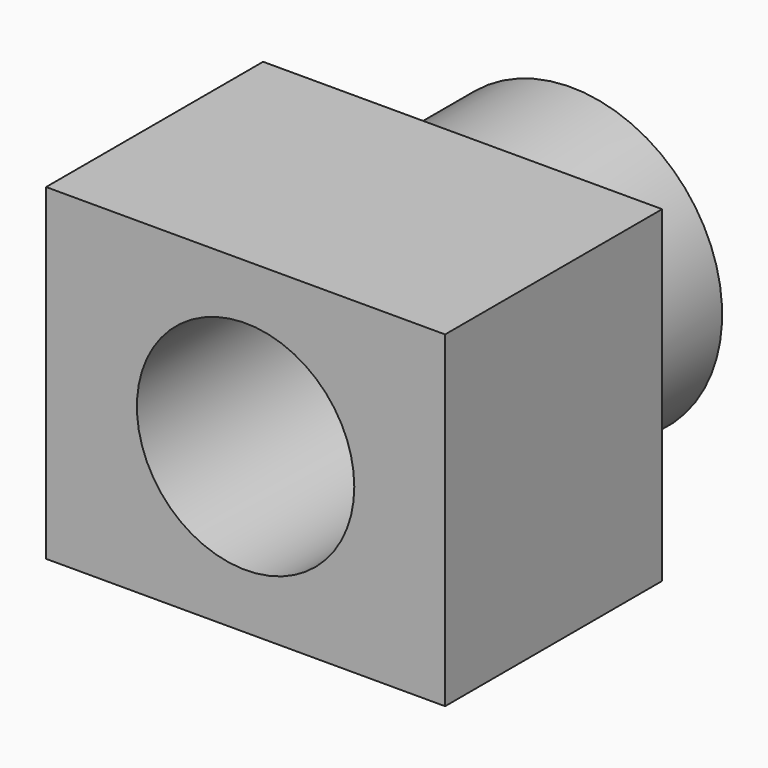
from build123d import *
from build123d import SkipClean  # not in build123d's __all__

# Parameters (mm, degrees)
F0_W     = 74.7220367193
F0_H     = 61.2964034081
F1_DEPTH = 25.4
F2_R     = 20.3537507695
F3_DEPTH = 50.801
F4_R     = 28.2811450825
F4_R_2   = 20.3537507695
F5_DEPTH = 25.4


with BuildPart() as f1:
    # F0 (on Front) → F1 (new body, symmetric)
    with BuildSketch(Plane.XZ):
        Rectangle(F0_W, F0_H)
    extrude(amount=F1_DEPTH, both=True)

    # F2 (on face) → F3 (cut, through all)
    with BuildSketch(Plane.XZ.offset(25.4)):
        Circle(F2_R)
    extrude(amount=-F3_DEPTH, mode=Mode.SUBTRACT)

    # F4 (on face) → F5 (join)
    with BuildSketch(Plane(origin=(0, 25.4, 0), x_dir=(-1, 0, 0), z_dir=(0, 1, 0))):
        Circle(F4_R)
        Circle(F4_R_2, mode=Mode.SUBTRACT)
    with SkipClean():  # cleaning this boolean's faces spoils the solid; the shape is the same uncleaned
        extrude(amount=F5_DEPTH)


solid = f1.part
